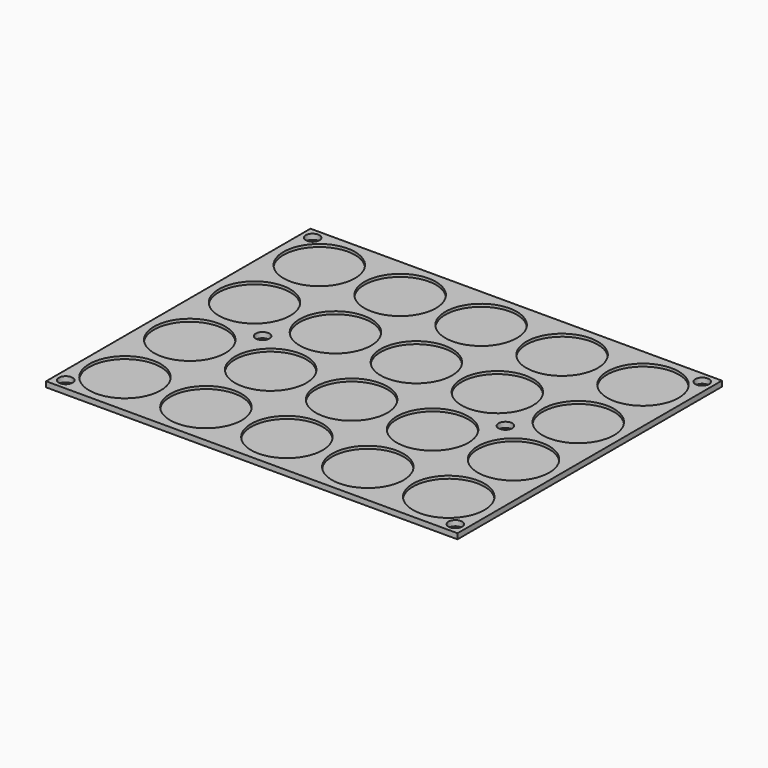
from build123d import *

# Parameters (mm, degrees)
F0_W     = 152.5
F0_H     = 122.5
F0_R     = 13.25
F1_DEPTH = 1
F2_DEPTH = 2
F3_R     = 2.55
F4_DEPTH = 2.001


# Not quite as in the source:
# - a feature names something its author has since deleted; it is built from what else it names


with BuildPart() as f1:
    # F0 (on Top) → F1 (new body)
    with BuildSketch(Plane.XY):
        Rectangle(F0_W, F0_H)
        with Locations((-60, -45)):
            Circle(F0_R, mode=Mode.SUBTRACT)
        with Locations((-30, -45)):
            Circle(F0_R, mode=Mode.SUBTRACT)
        with Locations((-60, -15)):
            Circle(F0_R, mode=Mode.SUBTRACT)
        with Locations((-30, -15)):
            Circle(F0_R, mode=Mode.SUBTRACT)
        with Locations((0, -45)):
            Circle(F0_R, mode=Mode.SUBTRACT)
        with Locations((30, -45)):
            Circle(F0_R, mode=Mode.SUBTRACT)
        with Locations((60, -45)):
            Circle(F0_R, mode=Mode.SUBTRACT)
        with Locations((0, -15)):
            Circle(F0_R, mode=Mode.SUBTRACT)
        with Locations((30, -15)):
            Circle(F0_R, mode=Mode.SUBTRACT)
        with Locations((60, -15)):
            Circle(F0_R, mode=Mode.SUBTRACT)
        with Locations((-60, 15)):
            Circle(F0_R, mode=Mode.SUBTRACT)
        with Locations((-30, 15)):
            Circle(F0_R, mode=Mode.SUBTRACT)
        with Locations((-60, 45)):
            Circle(F0_R, mode=Mode.SUBTRACT)
        with Locations((-30, 45)):
            Circle(F0_R, mode=Mode.SUBTRACT)
        with Locations((0, 15)):
            Circle(F0_R, mode=Mode.SUBTRACT)
        with Locations((30, 15)):
            Circle(F0_R, mode=Mode.SUBTRACT)
        with Locations((60, 15)):
            Circle(F0_R, mode=Mode.SUBTRACT)
        with Locations((0, 45)):
            Circle(F0_R, mode=Mode.SUBTRACT)
        with Locations((30, 45)):
            Circle(F0_R, mode=Mode.SUBTRACT)
        with Locations((60, 45)):
            Circle(F0_R, mode=Mode.SUBTRACT)
        with Locations((-60, 45)):
            Circle(F0_R)
        with Locations((-30, 45)):
            Circle(F0_R)
        with Locations((0, 45)):
            Circle(F0_R)
        with Locations((30, 45)):
            Circle(F0_R)
        with Locations((60, 45)):
            Circle(F0_R)
        with Locations((60, 15)):
            Circle(F0_R)
        with Locations((30, 15)):
            Circle(F0_R)
        with Locations((-30, 15)):
            Circle(F0_R)
        with Locations((-60, 15)):
            Circle(F0_R)
        with Locations((0, 15)):
            Circle(F0_R)
        with Locations((0, -15)):
            Circle(F0_R)
        with Locations((-30, -15)):
            Circle(F0_R)
        with Locations((-60, -15)):
            Circle(F0_R)
        with Locations((30, -15)):
            Circle(F0_R)
        with Locations((60, -15)):
            Circle(F0_R)
        with Locations((30, -45)):
            Circle(F0_R)
        with Locations((60, -45)):
            Circle(F0_R)
        with Locations((0, -45)):
            Circle(F0_R)
        with Locations((-30, -45)):
            Circle(F0_R)
        with Locations((-60, -45)):
            Circle(F0_R)
    extrude(amount=F1_DEPTH)

    # F0 (on Top) → F2 (join)
    with BuildSketch(Plane.XY):
        Rectangle(F0_W, F0_H)
        with Locations((-60, -45)):
            Circle(F0_R, mode=Mode.SUBTRACT)
        with Locations((-30, -45)):
            Circle(F0_R, mode=Mode.SUBTRACT)
        with Locations((-60, -15)):
            Circle(F0_R, mode=Mode.SUBTRACT)
        with Locations((-30, -15)):
            Circle(F0_R, mode=Mode.SUBTRACT)
        with Locations((0, -45)):
            Circle(F0_R, mode=Mode.SUBTRACT)
        with Locations((30, -45)):
            Circle(F0_R, mode=Mode.SUBTRACT)
        with Locations((60, -45)):
            Circle(F0_R, mode=Mode.SUBTRACT)
        with Locations((0, -15)):
            Circle(F0_R, mode=Mode.SUBTRACT)
        with Locations((30, -15)):
            Circle(F0_R, mode=Mode.SUBTRACT)
        with Locations((60, -15)):
            Circle(F0_R, mode=Mode.SUBTRACT)
        with Locations((-60, 15)):
            Circle(F0_R, mode=Mode.SUBTRACT)
        with Locations((-30, 15)):
            Circle(F0_R, mode=Mode.SUBTRACT)
        with Locations((-60, 45)):
            Circle(F0_R, mode=Mode.SUBTRACT)
        with Locations((-30, 45)):
            Circle(F0_R, mode=Mode.SUBTRACT)
        with Locations((0, 15)):
            Circle(F0_R, mode=Mode.SUBTRACT)
        with Locations((30, 15)):
            Circle(F0_R, mode=Mode.SUBTRACT)
        with Locations((60, 15)):
            Circle(F0_R, mode=Mode.SUBTRACT)
        with Locations((0, 45)):
            Circle(F0_R, mode=Mode.SUBTRACT)
        with Locations((30, 45)):
            Circle(F0_R, mode=Mode.SUBTRACT)
        with Locations((60, 45)):
            Circle(F0_R, mode=Mode.SUBTRACT)
    extrude(amount=F2_DEPTH)

    # F3 (on face) → F4 (cut, through all)
    with BuildSketch(Plane.XY.offset(2)):
        with Locations((-72.2, 57.2)):
            Circle(F3_R)
        with Locations((-45, 0)):
            Circle(F3_R)
        with Locations((72.2, 57.2)):
            Circle(F3_R)
        with Locations((45, 0)):
            Circle(F3_R)
        with Locations((72.2, -57.2)):
            Circle(F3_R)
        with Locations((-72.2, -57.2)):
            Circle(F3_R)
    extrude(amount=-F4_DEPTH, mode=Mode.SUBTRACT)


solid = f1.part
